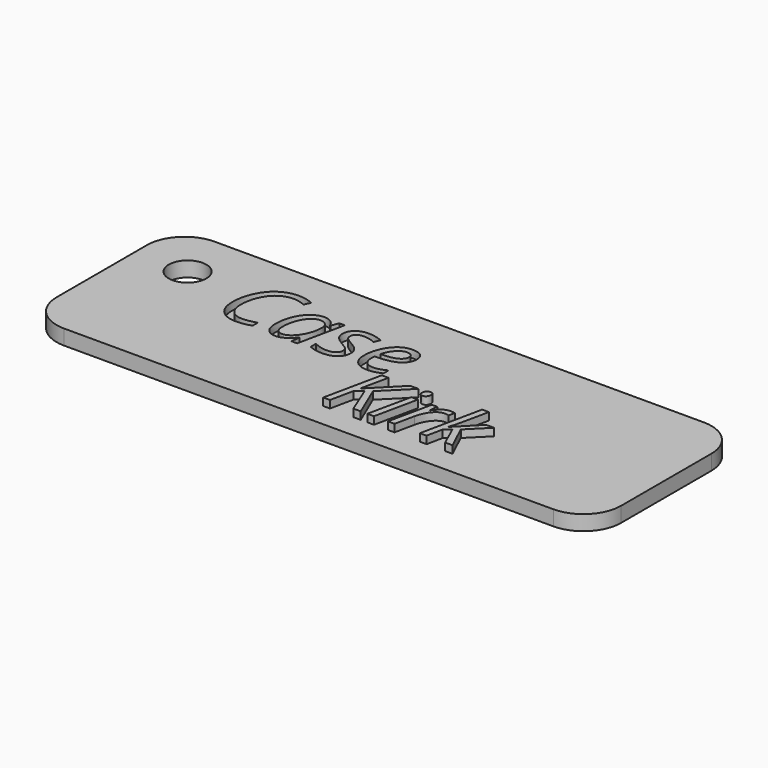
from build123d import *

# Parameters (mm, degrees)
F1_DEPTH     = 2
F3_D         = 5
F4_TEXT_SIZE = 11.6951479059
F5_DEPTH     = 1
F6_TEXT_SIZE = 10.7611485873
F7_DEPTH     = 1


# Not quite as in the source:
# - Text() gives the source's letters only with a copy of the font that has no kerning and outlines rounded to 1/6400 em; it was checked with that copy


with BuildPart() as f1:
    # F0 (on Top) → F1 (new body)
    with BuildSketch(Plane.XY):
        with BuildLine():
            ThreePointArc((37.5, 7.5), (36.0355339059, 11.0355339059), (32.5, 12.5))
            Line((32.5, 12.5), (-32.5, 12.5))
            ThreePointArc((-32.5, 12.5), (-36.0355339059, 11.0355339059), (-37.5, 7.5))
            Line((-37.5, 7.5), (-37.5, -7.5))
            ThreePointArc((-37.5, -7.5), (-36.0355339059, -11.0355339059), (-32.5, -12.5))
            Line((-32.5, -12.5), (32.5, -12.5))
            ThreePointArc((32.5, -12.5), (36.0355339059, -11.0355339059), (37.5, -7.5))
            Line((37.5, -7.5), (37.5, 7.5))
        make_face()
    extrude(amount=F1_DEPTH)

    # F3 (through all)
    with Locations(Plane.XY.offset(2)):
        with Locations((-30.5, 5.5)):
            Hole(F3_D / 2)

    # F4 (on face) → F5 (cut)
    with BuildSketch(Plane.XY.offset(2)):
        with Locations((-23.4548095614, 0)):
            Text('Case', F4_TEXT_SIZE, font='Open Sans', font_style=FontStyle.ITALIC, text_align=(TextAlign.LEFT, TextAlign.BOTTOM))
    extrude(amount=-F5_DEPTH, mode=Mode.SUBTRACT)

    # F6 (on face) → F7 (join)
    with BuildSketch(Plane.XY.offset(2)):
        with Locations((-1.0817694711, -9.3049267307)):
            Text('Kirk', F6_TEXT_SIZE, font='Open Sans', font_style=FontStyle.ITALIC, text_align=(TextAlign.LEFT, TextAlign.BOTTOM))
    extrude(amount=F7_DEPTH)


solid = f1.part
